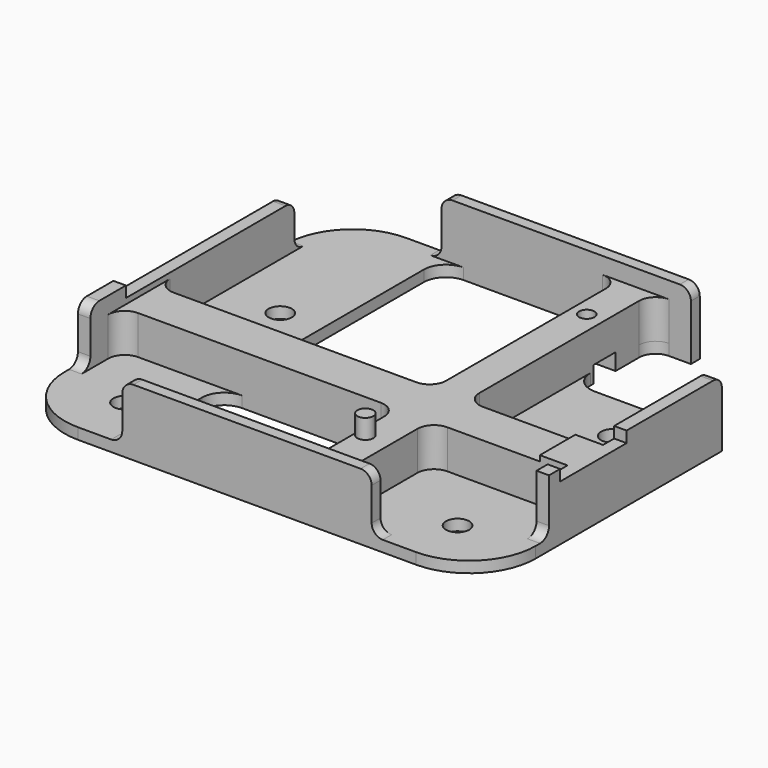
from build123d import *

# Parameters (mm, degrees)
F0_W      = 85
F0_H      = 74
F0_R      = 2.1
F1_DEPTH  = 12
F2_W      = 80.5
F2_H      = 70
F2_R      = 2.1
F3_DEPTH  = 10
F4_W      = 6
F4_H      = 42
F4_W_2    = 49.8
F4_H_2    = 8
F4_W_3    = 24.7
F4_H_3    = 20
F5_DEPTH  = 7
F6_R      = 1.45
F7_DEPTH  = 3.5
F8_W      = 2.25
F8_H      = 38
F9_DEPTH  = 2
F11_DEPTH = 10
F12_W     = 2.25
F12_H     = 15
F13_DEPTH = 2
F14_R     = 12
F15_R     = 3
F17_DEPTH = 2
F19_DEPTH = 2
F21_DEPTH = 2
F22_R     = 4
F23_R     = 2
F6_R_2    = 1.4
F24_DEPTH = 9
F25_W     = 6
F25_H     = 5
F25_R     = 1.4
F26_DEPTH = 3
F27_W     = 5
F27_H     = 8
F28_DEPTH = 1


with BuildPart() as f1:
    # F0 (on Top) → F1 (new body)
    with BuildSketch(Plane.XY):
        Rectangle(F0_W, F0_H)
        with Locations((-30, -27)):
            Circle(F0_R, mode=Mode.SUBTRACT)
        with Locations((30, -27)):
            Circle(F0_R, mode=Mode.SUBTRACT)
        with Locations((-30, 8)):
            Circle(F0_R, mode=Mode.SUBTRACT)
        with Locations((30, 8)):
            Circle(F0_R, mode=Mode.SUBTRACT)
    extrude(amount=F1_DEPTH)

    # F2 (on face) → F3 (cut)
    with BuildSketch(Plane.XY.offset(12)):
        Rectangle(F2_W, F2_H)
        with Locations((-30, -27)):
            Circle(F2_R, mode=Mode.SUBTRACT)
        with Locations((30, -27)):
            Circle(F2_R, mode=Mode.SUBTRACT)
        with Locations((-30, 8)):
            Circle(F2_R, mode=Mode.SUBTRACT)
        with Locations((30, 8)):
            Circle(F2_R, mode=Mode.SUBTRACT)
    extrude(amount=-F3_DEPTH, mode=Mode.SUBTRACT)

    # F4 (on face) → F5 (join)
    with BuildSketch(Plane.XY.offset(2)):
        with Locations((12.55, 14)):
            Rectangle(F4_W, F4_H)
        with Locations((-15.35, -11)):
            Rectangle(F4_W_2, F4_H_2)
        with Locations((12.55, -11)):
            Rectangle(F4_W, F4_H_2)
        with Locations((27.9, -11)):
            Rectangle(F4_W_3, F4_H_2)
        with Locations((12.55, -25)):
            Rectangle(F4_W, F4_H_3)
    extrude(amount=F5_DEPTH)

    # F6 (on face) → F7 (join)
    with BuildSketch(Plane.XY.offset(9)):
        with Locations((11.05, -24.1)):
            Circle(F6_R)
    extrude(amount=F7_DEPTH)

    # F8 (on face) → F9 (cut)
    with BuildSketch(Plane.XY.offset(12)):
        with Locations((-41.375, 5)):
            Rectangle(F8_W, F8_H)
    extrude(amount=-F9_DEPTH, mode=Mode.SUBTRACT)

    # F10 (on face) → F11 (cut, through all)
    with BuildSketch(Plane.XY.offset(12)):
        Polygon((-42.5, 37), (-42.5, 24), (-40.25, 24), (-40.25, 35), (-22.5, 35), (-22.5, 37), align=None)
        Polygon((42.5, 37), (22.5, 37), (22.5, 35), (40.25, 35), (40.25, 17), (42.5, 17), align=None)
        Polygon((42.5, -37), (42.5, -22), (40.25, -22), (40.25, -35), (22.5, -35), (22.5, -37), align=None)
        Polygon((-42.5, -37), (-22.5, -37), (-22.5, -35), (-40.25, -35), (-40.25, -22), (-42.5, -22), align=None)
    extrude(amount=-F11_DEPTH, mode=Mode.SUBTRACT)

    # F12 (on face) → F13 (cut)
    with BuildSketch(Plane.XY.offset(12)):
        with Locations((41.375, -12)):
            Rectangle(F12_W, F12_H)
    extrude(amount=-F13_DEPTH, mode=Mode.SUBTRACT)

    # F14
    f14_edges = [f1.edges().sort_by_distance(p)[0] for p in [
        (-42.5, 37, 1),
        (-42.5, -37, 1),
        (42.5, -37, 1),
        (42.5, 37, 1),
    ]]
    fillet(f14_edges, radius=F14_R)

    # F15
    f15_edges = [f1.edges().sort_by_distance(p)[0] for p in [
        (9.55, -7, 5.5),
        (9.55, -15, 5.5),
        (15.55, -15, 5.5),
        (15.55, -7, 5.5),
        (-40.25, -7, 5.5),
        (-40.25, -15, 5.5),
        (9.55, 35, 5.5),
        (15.55, 35, 5.5),
        (9.55, -35, 5.5),
        (40.25, -15, 5.5),
        (15.55, -35, 5.5),
    ]]
    fillet(f15_edges, radius=F15_R)

    # F16 (on face) → F17 (cut, through all)
    with BuildSketch(Plane.XY.offset(2)):
        with BuildLine():
            ThreePointArc((9.55, -18), (8.6713203436, -15.8786796564), (6.55, -15))
            Line((6.55, -15), (-22.5, -15))
            Line((-22.5, -15), (-22.5, -35))
            Line((-22.5, -35), (6.55, -35))
            ThreePointArc((6.55, -35), (8.6713203436, -34.1213203436), (9.55, -32))
            Line((9.55, -32), (9.55, -18))
        make_face()
    extrude(amount=-F17_DEPTH, mode=Mode.SUBTRACT)

    # F18 (on face) → F19 (cut, through all)
    with BuildSketch(Plane.XY.offset(2)):
        with BuildLine():
            Line((-22.5, 35), (-22.5, -7))
            Line((-22.5, -7), (6.55, -7))
            ThreePointArc((6.55, -7), (8.6713203436, -6.1213203436), (9.55, -4))
            Line((9.55, -4), (9.55, 32))
            ThreePointArc((9.55, 32), (8.6713203436, 34.1213203436), (6.55, 35))
            Line((6.55, 35), (-22.5, 35))
        make_face()
    extrude(amount=-F19_DEPTH, mode=Mode.SUBTRACT)

    # F20 (on face) → F21 (cut, through all)
    with BuildSketch(Plane.XY.offset(2)):
        with BuildLine():
            ThreePointArc((18.55, 35), (16.4286796564, 34.1213203436), (15.55, 32))
            Line((15.55, 32), (15.55, 17))
            Line((15.55, 17), (40.25, 17))
            Line((40.25, 17), (42.5, 17))
            Line((42.5, 17), (42.5, 25))
            ThreePointArc((42.5, 25), (38.9852813742, 33.4852813742), (30.5, 37))
            Line((30.5, 37), (22.5, 37))
            Line((22.5, 37), (22.5, 35))
            Line((22.5, 35), (18.55, 35))
        make_face()
    extrude(amount=-F21_DEPTH, mode=Mode.SUBTRACT)

    # F22
    f22_edges = [f1.edges().sort_by_distance(p)[0] for p in [
        (-22.5, 35, 1),
        (-22.5, -7, 1),
        (15.55, 17, 1),
        (-22.5, -15, 1),
        (-22.5, -35, 1),
    ]]
    fillet(f22_edges, radius=F22_R)

    # F23
    f23_edges = [f1.edges().sort_by_distance(p)[0] for p in [
        (-22.5, -36, 12),
        (22.5, -36, 12),
        (-41.375, -22, 12),
        (-22.5, 36, 12),
        (-22.5, 36, 2),
        (22.5, 36, 12),
        (41.375, 17, 12),
        (-41.375, 24, 10),
        (-22.5, -36, 2),
        (22.5, -36, 2),
        (41.375, -22, 2),
        (-41.375, -22, 2),
        (-41.375, 24, 2),
    ]]
    fillet(f23_edges, radius=F23_R)

    # F6 (on face) → F24 (cut, through all)
    with BuildSketch(Plane.XY.offset(9)):
        with Locations((12.35, 24.2)):
            Circle(F6_R_2)
    extrude(amount=-F24_DEPTH, mode=Mode.SUBTRACT)

    # F25 (on face) → F26 (cut)
    with BuildSketch(Plane(origin=(0, 0, 0), x_dir=(1, 0, 0), z_dir=(0, 0, -1))):
        with Locations((12.55, -24.2)):
            Rectangle(F25_W, F25_H)
        with Locations((12.35, -24.2)):
            Circle(F25_R, mode=Mode.SUBTRACT)
    extrude(amount=-F26_DEPTH, mode=Mode.SUBTRACT)

    # F27 (on face) → F28 (join, through all)
    with BuildSketch(Plane.XY.offset(9)):
        with Locations((37.75, -11)):
            Rectangle(F27_W, F27_H)
    extrude(amount=F28_DEPTH)


solid = f1.part
